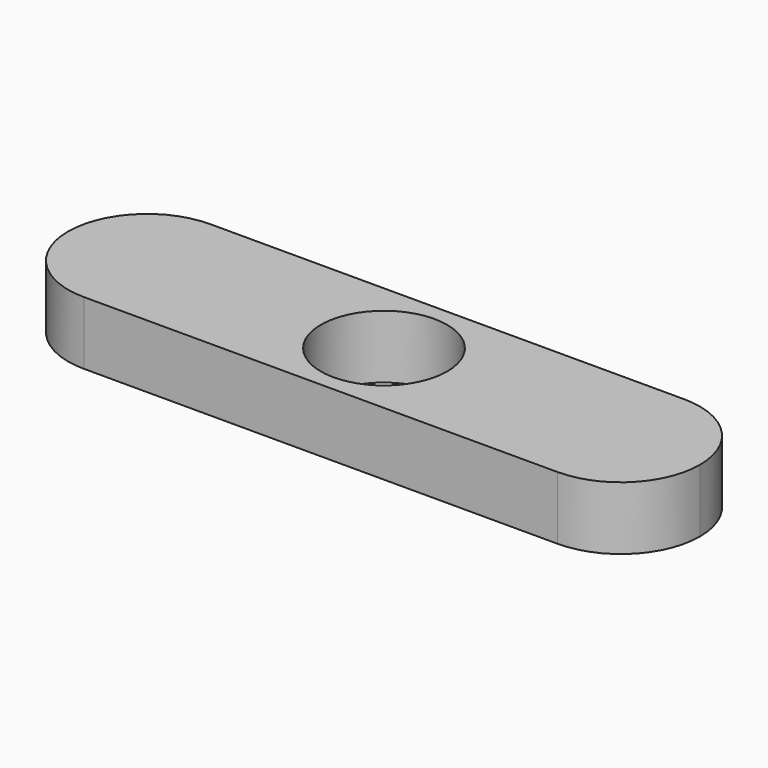
from build123d import *

# Parameters (mm, degrees)
F0_W     = 200
F0_H     = 50
F0_R     = 20
F1_DEPTH = 20
F2_R     = 24.99999


# Not quite as in the source:
# - a fillet or chamfer is up to 0.001 mm smaller than in the source, because OpenCascade refuses the exact size


with BuildPart() as f1:
    # F0 (on Top) → F1 (new body)
    with BuildSketch(Plane.XY):
        with Locations((100, 25)):
            Rectangle(F0_W, F0_H)
        with Locations((100, 25)):
            Circle(F0_R, mode=Mode.SUBTRACT)
    extrude(amount=F1_DEPTH)

    # F2 (radius 25 in the source; OpenCascade refuses exactly that, so slightly less here)
    f2_edges = [f1.edges().sort_by_distance(p)[0] for p in [
        (200, 0, 10),
        (200, 50, 10),
        (0, 50, 10),
        (0, 0, 10),
    ]]
    fillet(f2_edges, radius=F2_R)


solid = f1.part
